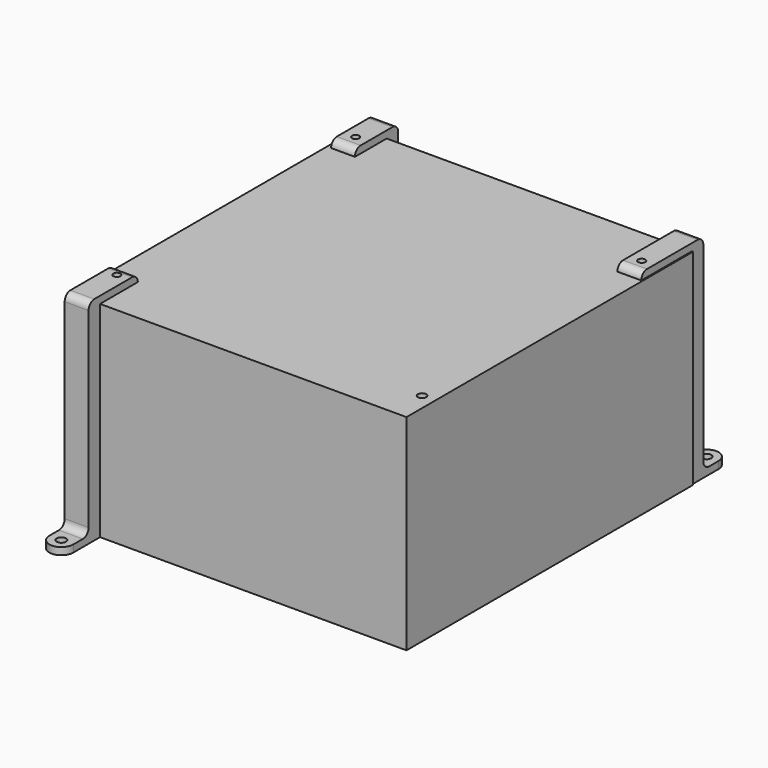
from build123d import *

# Parameters (mm, degrees)
F0_W      = 140
F0_H      = 150
F0_R      = 1.75
F1_DEPTH  = 86
F2_R      = 1.95
F3_DEPTH  = 3
F2_W      = 10
F2_H      = 6
F4_DEPTH  = 86
F5_W      = 10
F5_H      = 16.6205504089
F5_R      = 1.5
F5_H_2    = 6
F6_DEPTH  = 3
F7_R      = 1.95
F8_DEPTH  = 3
F7_W      = 10
F7_H      = 6
F9_DEPTH  = 86
F10_W     = 10
F10_H     = 32.4764741033
F10_R     = 1.5
F11_DEPTH = 3
F12_W     = 10
F12_H     = 6
F13_DEPTH = 86
F12_R     = 1.95
F14_DEPTH = 3
F15_W     = 10
F15_H     = 25.7673753845
F15_R     = 1.5
F16_DEPTH = 3
F17_R     = 2.99999
F17_2_R   = 2.99999
F17_3_R   = 2.99999


# Not quite as in the source:
# - a fillet or chamfer is up to 0.001 mm smaller than in the source, because OpenCascade refuses the exact size


with BuildPart() as f1:
    # F0 (on Top) → F1 (new body)
    with BuildSketch(Plane.XY):
        Rectangle(F0_W, F0_H)
        with Locations((-63.3, -60)):
            Circle(F0_R, mode=Mode.SUBTRACT)
        with Locations((64.5, -60)):
            Circle(F0_R, mode=Mode.SUBTRACT)
        with Locations((-63.3, 65)):
            Circle(F0_R, mode=Mode.SUBTRACT)
        with Locations((64.5, 55)):
            Circle(F0_R, mode=Mode.SUBTRACT)
    extrude(amount=F1_DEPTH)


with BuildPart() as f3:
    # F2 (on Top) → F3 (new body)
    with BuildSketch(Plane.XY):
        with BuildLine():
            ThreePointArc((-68.3, 89), (-63.3, 84), (-58.3, 89))
            ThreePointArc((-58.3, 89), (-63.3, 94), (-68.3, 89))
        make_face()
        with Locations((-63.3, 89)):
            Circle(F2_R, mode=Mode.SUBTRACT)
        with BuildLine():
            Line((-58.3, 81), (-58.3, 89))
            ThreePointArc((-58.3, 89), (-63.3, 84), (-68.3, 89))
            Line((-68.3, 89), (-68.3, 81))
            Line((-68.3, 81), (-58.3, 81))
        make_face()
    extrude(amount=F3_DEPTH)

    # F2 (on Top) → F4 (join)
    with BuildSketch(Plane.XY):
        with Locations((-63.3, 78)):
            Rectangle(F2_W, F2_H)
    extrude(amount=F4_DEPTH)

    # F5 (on face) → F6 (join)
    with BuildSketch(Plane.XY.offset(86)):
        with Locations((-63.3, 66.6897247956)):
            Rectangle(F5_W, F5_H)
        with Locations((-63.3, 65)):
            Circle(F5_R, mode=Mode.SUBTRACT)
        with Locations((-63.3, 78)):
            Rectangle(F5_W, F5_H_2)
    extrude(amount=F6_DEPTH)

    # F17 (radius 3 in the source; OpenCascade refuses exactly that, so slightly less here)
    f17_edges = [f3.edges().sort_by_distance(p)[0] for p in [
        (-63.3, 81, 89),
        (-63.3, 81, 3),
        (-63.3, 58.37945, 89),
    ]]
    fillet(f17_edges, radius=F17_R)


with BuildPart() as f8:
    # F7 (on Top) → F8 (new body)
    with BuildSketch(Plane.XY):
        with BuildLine():
            ThreePointArc((59.5, 89), (64.5, 84), (69.5, 89))
            ThreePointArc((69.5, 89), (64.5, 94), (59.5, 89))
        make_face()
        with Locations((64.5, 89)):
            Circle(F7_R, mode=Mode.SUBTRACT)
        with BuildLine():
            Line((69.5, 81), (69.5, 89))
            ThreePointArc((69.5, 89), (64.5, 84), (59.5, 89))
            Line((59.5, 89), (59.5, 81))
            Line((59.5, 81), (69.5, 81))
        make_face()
    extrude(amount=F8_DEPTH)

    # F7 (on Top) → F9 (join)
    with BuildSketch(Plane.XY):
        with Locations((64.5, 78)):
            Rectangle(F7_W, F7_H)
    extrude(amount=F9_DEPTH)

    # F10 (on face) → F11 (join)
    with BuildSketch(Plane.XY.offset(86)):
        with Locations((64.5, 64.7617629484)):
            Rectangle(F10_W, F10_H)
        with Locations((64.5, 55)):
            Circle(F10_R, mode=Mode.SUBTRACT)
    extrude(amount=F11_DEPTH)

    # F17#2 (radius 3 in the source; OpenCascade refuses exactly that, so slightly less here)
    f17_2_edges = [f8.edges().sort_by_distance(p)[0] for p in [
        (64.5, 81, 89),
        (64.5, 81, 3),
        (64.5, 48.523526, 89),
    ]]
    fillet(f17_2_edges, radius=F17_2_R)


with BuildPart() as f13:
    # F12 (on Top) → F13 (new body)
    with BuildSketch(Plane.XY):
        with Locations((-63.3374598043, -78)):
            Rectangle(F12_W, F12_H)
    extrude(amount=F13_DEPTH)

    # F12 (on Top) → F14 (join)
    with BuildSketch(Plane.XY):
        with BuildLine():
            ThreePointArc((-68.3374598043, -89), (-63.3374598043, -84), (-58.3374598043, -89))
            Line((-58.3374598043, -89), (-58.3374598043, -81))
            Line((-58.3374598043, -81), (-68.3374598043, -81))
            Line((-68.3374598043, -81), (-68.3374598043, -89))
        make_face()
        with BuildLine():
            ThreePointArc((-68.3374598043, -89), (-63.3374598043, -94), (-58.3374598043, -89))
            ThreePointArc((-58.3374598043, -89), (-63.3374598043, -84), (-68.3374598043, -89))
        make_face()
        with Locations((-63.3374598043, -89)):
            Circle(F12_R, mode=Mode.SUBTRACT)
    extrude(amount=F14_DEPTH)

    # F15 (on face) → F16 (join)
    with BuildSketch(Plane.XY.offset(86)):
        with Locations((-63.3374598043, -68.1163123077)):
            Rectangle(F15_W, F15_H)
        with Locations((-63.3, -60)):
            Circle(F15_R, mode=Mode.SUBTRACT)
    extrude(amount=F16_DEPTH)

    # F17#3 (radius 3 in the source; OpenCascade refuses exactly that, so slightly less here)
    f17_3_edges = [f13.edges().sort_by_distance(p)[0] for p in [
        (-63.33746, -81, 89),
        (-63.33746, -55.232625, 89),
        (-63.33746, -81, 3),
    ]]
    fillet(f17_3_edges, radius=F17_3_R)


solid = Compound([f1.part, f3.part, f8.part, f13.part])
